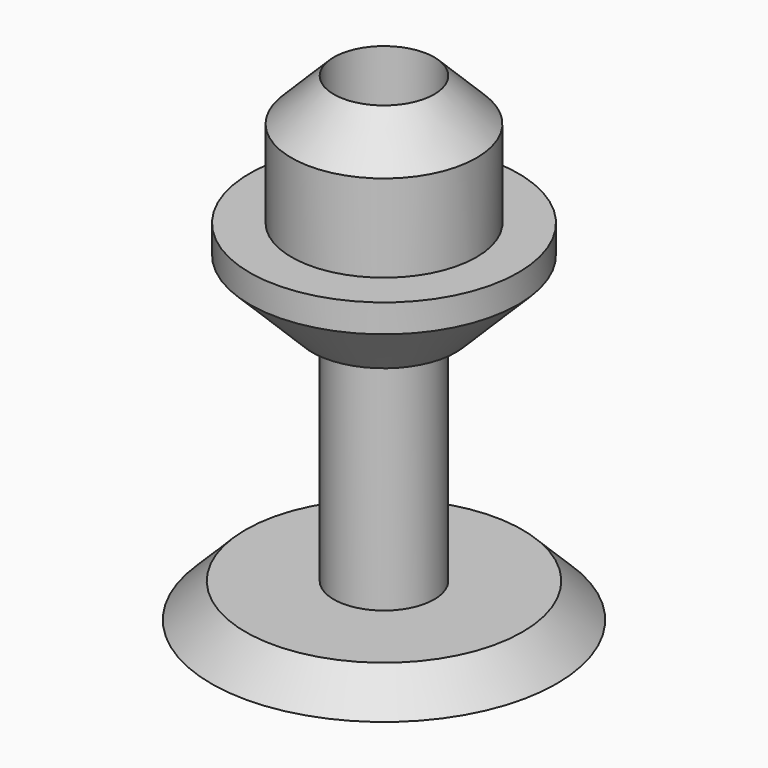
from build123d import *

# Parameters (mm, degrees)
F0_R      = 16.354359017
F1_DEPTH  = 2.794
F5_R      = 4.0904887837
F6_DEPTH  = 18.288
F7_R      = 7.5325975951
F7_R_2    = 4.0904887837
F8_DEPTH  = 19.558
F10_R     = 10.9404048471
F10_R_2   = 4.0904887837
F11_DEPTH = 7.366
F12_SIZE  = 5.08


# Not quite as in the source:
# - a fillet or chamfer that OpenCascade refuses, or shapes differently, is made with other operations: its cross-section is extruded or revolved along the edge and cut away or added
# - the program builds the solid bodies; features that only make, move or delete a surface that nothing else refers to are left out


with BuildPart() as f1:
    # F0 (on Top) → F1 (new body)
    with BuildSketch(Plane.XY):
        Circle(F0_R)
    extrude(amount=F1_DEPTH)

    # F2: chamfer of 5.08 on 1 edges, made by hand

    # F2_s1 → F2_t2 (revolve, cut)
    with BuildSketch(Plane.XZ):
        Polygon((16.354359017, -2.286), (11.274359017, 2.794), (16.354359017, 2.794), align=None)
    revolve(axis=Axis((0, 0, 2.794), (0, 0, 1)), mode=Mode.SUBTRACT)

    # F5 (on face) → F6 (join)
    with BuildSketch(Plane.XY.offset(2.794)):
        Circle(F5_R)
    extrude(amount=F6_DEPTH)


with BuildPart() as f8:
    # F7 (on face) → F8 (new body)
    with BuildSketch(Plane.XY.offset(21.082)):
        Circle(F7_R)
        Circle(F7_R_2, mode=Mode.SUBTRACT)
    extrude(amount=F8_DEPTH)

    # F9: chamfer of 5.08 on 1 edges, made by hand

    # F9_s1 → F9_t2 (revolve, cut)
    with BuildSketch(Plane.XZ):
        Polygon((7.5325975951, 35.56), (2.4525975951, 40.64), (7.5325975951, 40.64), align=None)
    revolve(axis=Axis((0, 0, 40.64), (0, 0, 1)), mode=Mode.SUBTRACT)

    # F10 (on face) → F11 (join)
    with BuildSketch(Plane.XY.offset(21.082)):
        Circle(F10_R)
        Circle(F10_R_2, mode=Mode.SUBTRACT)
    extrude(amount=F11_DEPTH)

    # F12
    f12_edges = [f8.edges().sort_by_distance(p)[0] for p in [
        (-10.940405, 0, 21.082),
    ]]
    chamfer(f12_edges, length=F12_SIZE)


solid = Compound([f1.part, f8.part])
